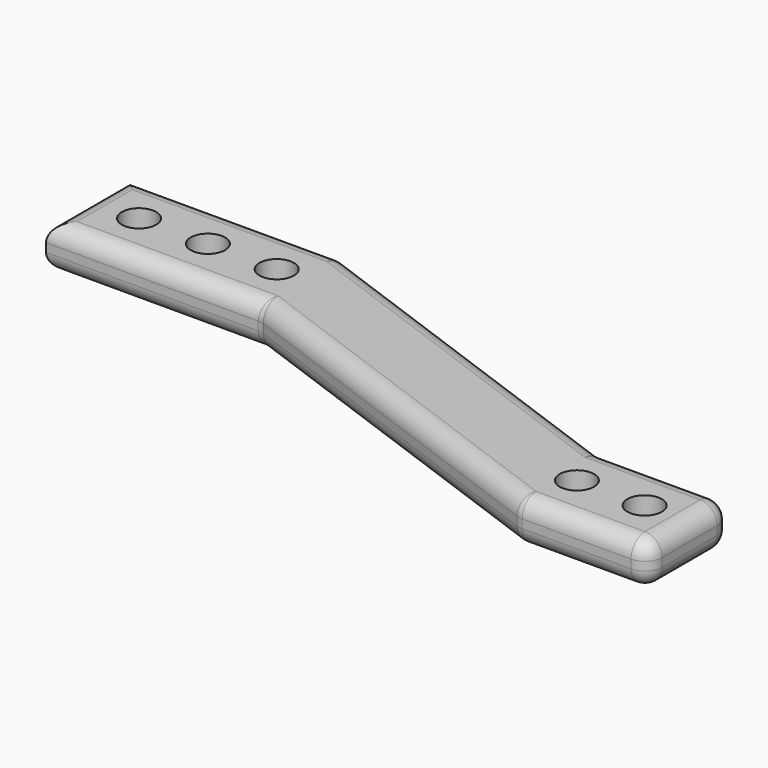
from build123d import *

# Parameters (mm, degrees)
F0_W         = 25
F0_H         = 12
F0_R         = 2
F1_DEPTH     = 5
F2_R         = 2
F3_R         = 2
F4_R         = 2
F5_R         = 2
F6_T1_DEPTH  = 1
F6_T6_DEPTH  = 2
F6_T12_DEPTH = 2
F6_S17_W     = 2
F6_S17_H     = 2
F6_T18_DEPTH = 2
F6_S23_W     = 2
F6_S23_H     = 2
F6_T24_DEPTH = 2
F7_T1_DEPTH  = 1
F7_S5_W      = 2
F7_S5_H      = 2
F7_T6_DEPTH  = 2
F7_S11_W     = 2
F7_S11_H     = 2
F7_T12_DEPTH = 2
F8_R         = 2


# Not quite as in the source:
# - a fillet or chamfer that OpenCascade refuses, or shapes differently, is made with other operations: its cross-section is extruded or revolved along the edge and cut away or added


with BuildPart() as f1:
    # F0 (on Top) → F1 (new body)
    with BuildSketch(Plane.XY):
        with Locations((-12.5, 6)):
            Rectangle(F0_W, F0_H)
        with Locations((-19, 6)):
            Circle(F0_R, mode=Mode.SUBTRACT)
        with Locations((-11, 6)):
            Circle(F0_R, mode=Mode.SUBTRACT)
        with Locations((-3, 6)):
            Circle(F0_R, mode=Mode.SUBTRACT)
        Polygon((0, 12), (0, 0), (42.2861679354, -15.3909064497), (57.2861679354, -15.3909064497), (57.2861679354, -3.3909064497), (42.2861679354, -3.3909064497), align=None)
        with Locations((44.1906489432, -9.3909064497)):
            Circle(F0_R, mode=Mode.SUBTRACT)
        with Locations((52.0649450129, -9.3909064497)):
            Circle(F0_R, mode=Mode.SUBTRACT)
    extrude(amount=F1_DEPTH)

    # F2
    f2_edges = [f1.edges().sort_by_distance(p)[0] for p in [
        (-12.5, 0, 0),
        (-25, 6, 0),
        (-12.5, 12, 0),
        (21.143084, 4.304547, 0),
        (49.786168, -3.390906, 0),
        (57.286168, -9.390906, 0),
        (49.786168, -15.390906, 0),
        (21.143084, -7.695453, 0),
    ]]
    fillet(f2_edges, radius=F2_R)

    # F3
    f3_edges = [f1.edges().sort_by_distance(p)[0] for p in [
        (57.286168, -9.390906, 5),
        (49.786168, -15.390906, 5),
        (21.143084, -7.695453, 5),
        (-12.5, 0, 5),
        (-25, 6, 5),
        (-12.5, 12, 5),
        (21.143084, 4.304547, 5),
        (49.786168, -3.390906, 5),
    ]]
    fillet(f3_edges, radius=F3_R)

    # F4
    f4_edges = [f1.edges().sort_by_distance(p)[0] for p in [
        (42.181922, -3.982115, 4.419615),
        (42.286168, -3.390906, 2.5),
        (42.181922, -3.982115, 0.580385),
    ]]
    fillet(f4_edges, radius=F4_R)

    # F5
    f5_edges = [f1.edges().sort_by_distance(p)[0] for p in [
        (0.104246, 0.591209, 4.419615),
        (0, 0, 2.5),
        (0.104246, 0.591209, 0.580385),
    ]]
    fillet(f5_edges, radius=F5_R)

    # F6: fillet of radius 2 on 6 edges, made by hand

    # F6_s2 → F6_t1 (cut)
    with BuildSketch(Plane.XY.offset(2)):
        with BuildLine():
            ThreePointArc((41.9547816101, -15.2702916912), (42.2915255414, -15.3605219557), (42.6388218968, -15.3909064497))
            Line((42.6388218968, -15.3909064497), (42.2861679354, -15.3909064497))
            Line((42.2861679354, -15.3909064497), (41.9547816101, -15.2702916912))
        make_face()
        with BuildLine():
            ThreePointArc((55.2861679354, -15.3909064497), (56.7003814977, -14.805120012), (57.2861679354, -13.3909064497))
            Line((57.2861679354, -13.3909064497), (57.2861679354, -15.3909064497))
            Line((57.2861679354, -15.3909064497), (55.2861679354, -15.3909064497))
        make_face()
    extrude(amount=F6_T1_DEPTH, mode=Mode.SUBTRACT)


with BuildPart() as f6_tool4:
    # F6_s5 → F6_t6 (new body)
    with BuildSketch(Plane.XY.offset(3)):
        Polygon((42.6388218968, -13.3909064497), (41.9547816101, -15.2702916912), (42.2861679354, -15.3909064497), (42.6388218968, -15.3909064497), align=None)
    extrude(amount=F6_T6_DEPTH)

    # F6_s7 → F6_t8 (revolve, cut)
    with BuildSketch(Plane(origin=(42.6388218968, -13.3909064497, 3), x_dir=(0.1736481777, 0.984807753, 0), z_dir=(0.984807753, -0.1736481777, 0))):
        with BuildLine():
            ThreePointArc((0, -2), (2, 0), (0, 2))
            Line((0, 2), (0, -2))
        make_face()
    revolve(axis=Axis((42.6388218968, -13.3909064497, 3), (0, 0, 1)), mode=Mode.SUBTRACT)


with BuildPart() as f1_1:
    add(f1.part)

    # F6_t3: cut F6_tool4
    add(f6_tool4.part, mode=Mode.SUBTRACT)


with BuildPart() as f6_tool10:
    # F6_s11 → F6_t12 (new body)
    with BuildSketch(Plane.XY.offset(2)):
        Polygon((42.6388218968, -13.3909064497), (41.9547816101, -15.2702916912), (42.2861679354, -15.3909064497), (42.6388218968, -15.3909064497), align=None)
    extrude(amount=-F6_T12_DEPTH)

    # F6_s13 → F6_t14 (revolve, cut)
    with BuildSketch(Plane(origin=(42.6388218968, -13.3909064497, 2), x_dir=(0.1736481777, 0.984807753, 0), z_dir=(-0.984807753, 0.1736481777, 0))):
        with BuildLine():
            ThreePointArc((0, -2), (2, 0), (0, 2))
            Line((0, 2), (0, -2))
        make_face()
    revolve(axis=Axis((42.6388218968, -13.3909064497, 2), (0, 0, -1)), mode=Mode.SUBTRACT)


with BuildPart() as f1_2:
    add(f1_1.part)

    # F6_t9: cut F6_tool10
    add(f6_tool10.part, mode=Mode.SUBTRACT)


with BuildPart() as f6_tool16:
    # F6_s17 → F6_t18 (new body)
    with BuildSketch(Plane.XZ.offset(13.3909064497)):
        with Locations((56.2861679354, 4)):
            Rectangle(F6_S17_W, F6_S17_H)
    extrude(amount=F6_T18_DEPTH)

    # F6_s19 → F6_t20 (revolve, cut)
    with BuildSketch(Plane(origin=(55.2861679354, -13.3909064497, 3), x_dir=(-0.7071067812, 0, -0.7071067812), z_dir=(-0.7071067812, 0, 0.7071067812))):
        with BuildLine():
            ThreePointArc((0, -2), (2, 0), (0, 2))
            Line((0, 2), (0, -2))
        make_face()
    revolve(axis=Axis((55.2861679354, -13.3909064497, 3), (0, -1, 0)), mode=Mode.SUBTRACT)


with BuildPart() as f1_3:
    add(f1_2.part)

    # F6_t15: cut F6_tool16
    add(f6_tool16.part, mode=Mode.SUBTRACT)


with BuildPart() as f6_tool22:
    # F6_s23 → F6_t24 (new body)
    with BuildSketch(Plane.XZ.offset(13.3909064497)):
        with Locations((56.2861679354, 1)):
            Rectangle(F6_S23_W, F6_S23_H)
    extrude(amount=F6_T24_DEPTH)

    # F6_s25 → F6_t26 (revolve, cut)
    with BuildSketch(Plane(origin=(55.2861679354, -13.3909064497, 2), x_dir=(-0.7071067812, 0, 0.7071067812), z_dir=(0.7071067812, 0, 0.7071067812))):
        with BuildLine():
            ThreePointArc((0, -2), (2, 0), (0, 2))
            Line((0, 2), (0, -2))
        make_face()
    revolve(axis=Axis((55.2861679354, -13.3909064497, 2), (0, -1, 0)), mode=Mode.SUBTRACT)


with BuildPart() as f1_4:
    add(f1_3.part)

    # F6_t21: cut F6_tool22
    add(f6_tool22.part, mode=Mode.SUBTRACT)

    # F7: fillet of radius 2 on 3 edges, made by hand

    # F7_s2 → F7_t1 (cut)
    with BuildSketch(Plane.XY.offset(2)):
        with BuildLine():
            ThreePointArc((57.2861679354, -5.3909064497), (56.7003814977, -3.9766928873), (55.2861679354, -3.3909064497))
            Line((55.2861679354, -3.3909064497), (57.2861679354, -3.3909064497))
            Line((57.2861679354, -3.3909064497), (57.2861679354, -5.3909064497))
        make_face()
    extrude(amount=F7_T1_DEPTH, mode=Mode.SUBTRACT)


with BuildPart() as f7_tool4:
    # F7_s5 → F7_t6 (new body)
    with BuildSketch(Plane.YZ.offset(55.2861679354)):
        with Locations((-4.3909064497, 4)):
            Rectangle(F7_S5_W, F7_S5_H)
    extrude(amount=F7_T6_DEPTH)

    # F7_s7 → F7_t8 (revolve, cut)
    with BuildSketch(Plane(origin=(55.2861679354, -5.3909064497, 3), x_dir=(0, -0.7071067812, -0.7071067812), z_dir=(0, -0.7071067812, 0.7071067812))):
        with BuildLine():
            ThreePointArc((0, -2), (2, 0), (0, 2))
            Line((0, 2), (0, -2))
        make_face()
    revolve(axis=Axis((55.2861679354, -5.3909064497, 3), (1, 0, 0)), mode=Mode.SUBTRACT)


with BuildPart() as f1_5:
    add(f1_4.part)

    # F7_t3: cut F7_tool4
    add(f7_tool4.part, mode=Mode.SUBTRACT)


with BuildPart() as f7_tool10:
    # F7_s11 → F7_t12 (new body)
    with BuildSketch(Plane.YZ.offset(55.2861679354)):
        with Locations((-4.3909064497, 1)):
            Rectangle(F7_S11_W, F7_S11_H)
    extrude(amount=F7_T12_DEPTH)

    # F7_s13 → F7_t14 (revolve, cut)
    with BuildSketch(Plane(origin=(55.2861679354, -5.3909064497, 2), x_dir=(0, -0.7071067812, 0.7071067812), z_dir=(0, 0.7071067812, 0.7071067812))):
        with BuildLine():
            ThreePointArc((0, -2), (2, 0), (0, 2))
            Line((0, 2), (0, -2))
        make_face()
    revolve(axis=Axis((55.2861679354, -5.3909064497, 2), (1, 0, 0)), mode=Mode.SUBTRACT)


with BuildPart() as f1_6:
    add(f1_5.part)

    # F7_t9: cut F7_tool10
    add(f7_tool10.part, mode=Mode.SUBTRACT)

    # F8
    f8_edges = [f1_6.edges().sort_by_distance(p)[0] for p in [
        (-0.104246, 11.408791, 0.580385),
        (-0.104246, 11.408791, 4.419615),
        (0, 12, 2.5),
    ]]
    fillet(f8_edges, radius=F8_R)


solid = f1_6.part
